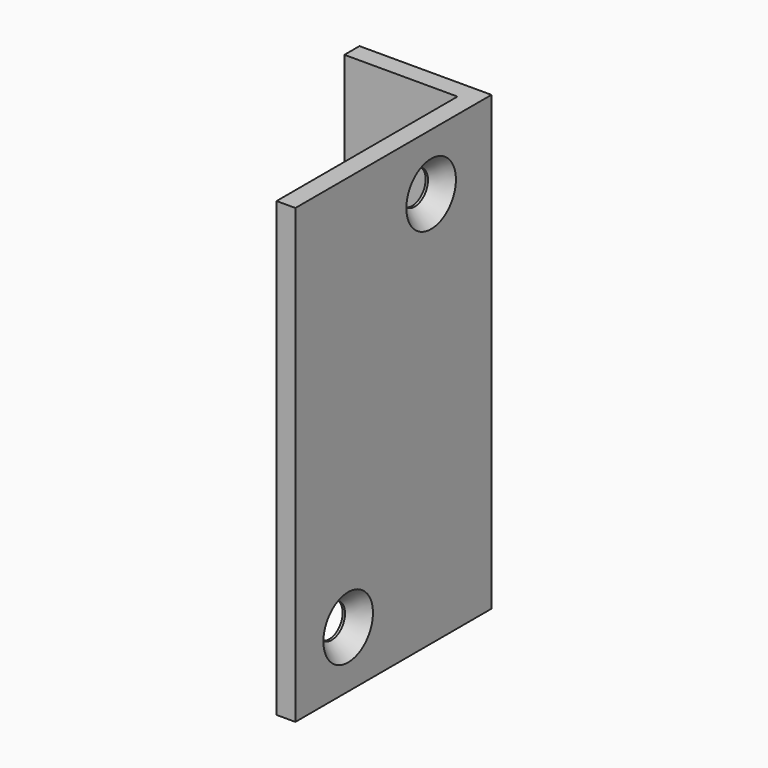
from build123d import *

# Parameters (mm, degrees)
F0_W           = 41.275
F0_H           = 76.2
F1_DEPTH       = 22.225
F3_D           = 5.6134
F3_CSINK_D     = 10.4394
F3_CSINK_ANGLE = 82
F4_W           = 19.05
F4_H           = 38.1
F5_DEPTH       = 76.201


# Not quite as in the source:
# - a feature names something its author has since deleted; it is built from what else it names


with BuildPart() as f1:
    # F0 (on Right) → F1 (new body)
    with BuildSketch(Plane.YZ):
        Rectangle(F0_W, F0_H)
    extrude(amount=F1_DEPTH)

    # F3 (through all)
    with Locations(Plane.YZ.offset(22.225)):
        with Locations((7.9375, 28.575), (-9.525, -28.575)):
            CounterSinkHole(F3_D / 2, F3_CSINK_D / 2, counter_sink_angle=F3_CSINK_ANGLE)

    # F4 (on face) → F5 (cut, through all)
    with BuildSketch(Plane.XY.offset(38.1)):
        with Locations((9.525, -1.5875)):
            Rectangle(F4_W, F4_H)
    extrude(amount=-F5_DEPTH, mode=Mode.SUBTRACT)


solid = f1.part
